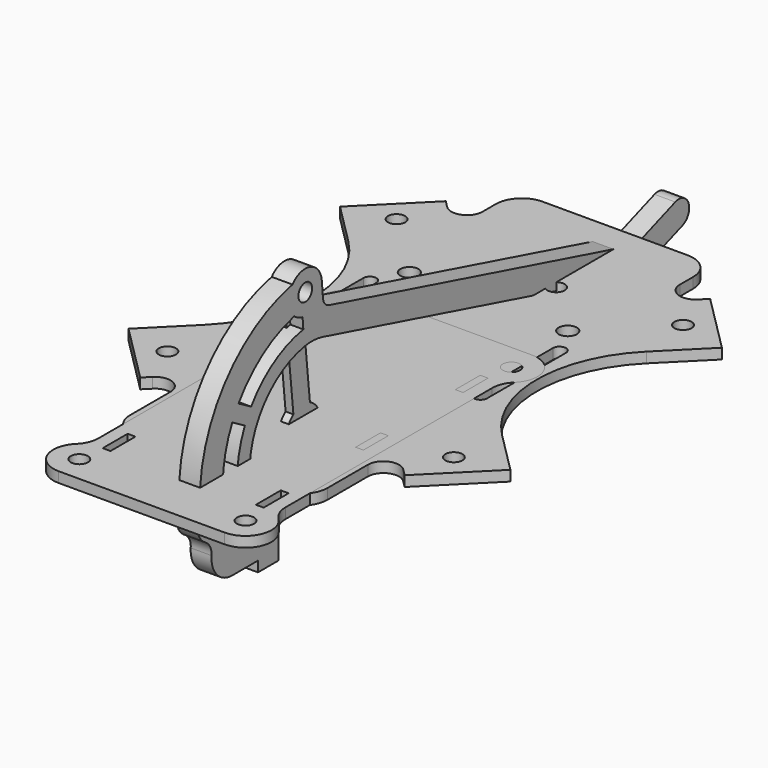
from build123d import *

# Parameters (mm, degrees)
F0_R      = 1.65
F1_DEPTH  = 4
F2_R      = 2
F3_R      = 1.65
F3_R_2    = 1.5
F4_DEPTH  = 1.5
F5_W      = 4
F5_H      = 5
F5_R      = 1.65
F5_R_2    = 1.75
F6_DEPTH  = 2
F7_R      = 1.5
F8_DEPTH  = 1.5
F9_R      = 1.65
F9_W      = 1.5
F9_H      = 6
F10_DEPTH = 2


with BuildPart() as f1:
    # F0 (on Right) → F1 (new body)
    with BuildSketch(Plane.YZ):
        with BuildLine():
            ThreePointArc((1.3715672107, 25.2116703552), (-1.4222724525, 28.6816418888), (-5.6933412888, 27.4150663864))
            ThreePointArc((-5.6933412888, 27.4150663864), (-22.1102697021, 17.1795219288), (-27.9717466489, -1.2575330657))
            ThreePointArc((-27.9717466489, -1.2575330657), (-28.0255548079, -1.9734585405), (-28.2479227846, -2.6560983329))
            ThreePointArc((-28.2479227846, -2.6560983329), (-28.4395274813, -5.5297709835), (-26.6511163601, -7.7872679434))
            ThreePointArc((-26.6511163601, -7.7872679434), (-25.5130767857, -8.9869520262), (-25.183571367, -10.607384731))
            ThreePointArc((-25.183571367, -10.607384731), (-23.8707312949, -14.3938859479), (-20.1990098767, -16))
            Line((-20.1990098767, -16), (-14, -16))
            Line((-14, -16), (-14, -18))
            Line((-14, -18), (-9, -18))
            Line((-9, -18), (-9, -16))
            Line((-9, -16), (-9, -13.7477270849))
            ThreePointArc((-9, -13.7477270849), (-9.1088672113, -13.2939844784), (-9.4117647059, -12.9390372563))
            ThreePointArc((-9.4117647059, -12.9390372563), (-11.0490391197, -11.5723262369), (-12.4899959968, -10))
            ThreePointArc((-12.4899959968, -10), (-14.9520494126, 5.6952803585), (-2.6721102867, 15.7752916491))
            ThreePointArc((-2.6721102867, 15.7752916491), (-0.5321831807, 15.9046899341), (1.5861490935, 15.5749926313))
            Line((1.5861490935, 15.5749926313), (77.2740661031, -4.7055236082))
            Line((77.2740661031, -4.7055236082), (88.1524135642, -0.7461289344))
            ThreePointArc((88.1524135642, -0.7461289344), (89.6465947578, 2.4581529759), (86.4423128475, 3.9523341695))
            Line((86.4423128475, 3.9523341695), (78.2305224207, 0.9634868841))
            ThreePointArc((78.2305224207, 0.9634868841), (77.0369193968, 0.726064481), (75.827165667, 0.8585540621))
            Line((75.827165667, 0.8585540621), (3.1187059905, 20.3407271153))
            ThreePointArc((3.1187059905, 20.3407271153), (2.1042551945, 20.9870035486), (1.6439546845, 22.0982672824))
            Line((1.6439546845, 22.0982672824), (1.3715672107, 25.2116703552))
        make_face()
        with Locations((-24.6201938253, -4.3412044417)):
            Circle(F0_R, mode=Mode.SUBTRACT)
        with BuildLine():
            Line((-16.1554944214, -10), (-20.1556443707, -10))
            ThreePointArc((-20.1556443707, -10), (-20.8662969598, -8.4171046796), (-21.4528611452, -6.7841542351))
            ThreePointArc((-21.4528611452, -6.7841542351), (-20.6244591351, -4.1565309852), (-21.6916970528, -1.6165197528))
            ThreePointArc((-21.6916970528, -1.6165197528), (-22.2990522616, -0.640297429), (-22.4946051617, 0.4926851121))
            ThreePointArc((-22.4946051617, 0.4926851121), (-21.8583588524, 5.3349928099), (-20.1922220952, 9.9259340546))
            Line((-20.1922220952, 9.9259340546), (-17.1531247023, 8.1713103568))
            ThreePointArc((-17.1531247023, 8.1713103568), (-18.97143002, -1.0415579663), (-16.1554944214, -10))
        make_face(mode=Mode.SUBTRACT)
        with BuildLine():
            ThreePointArc((-18.6922220952, 12.524010266), (-12.8614022088, 18.4616990882), (-5.2711524312, 21.8738417304))
            ThreePointArc((-5.2711524312, 21.8738417304), (-4.3390469936, 21.2545169172), (-3.2718535396, 20.9176461662))
            Line((-3.2718535396, 20.9176461662), (-3.0820652908, 18.7483565558))
            ThreePointArc((-3.0820652908, 18.7483565558), (-10.181739858, 16.0415764021), (-15.6531247023, 10.7693865681))
            Line((-15.6531247023, 10.7693865681), (-18.6922220952, 12.524010266))
        make_face(mode=Mode.SUBTRACT)
        with Locations((-2.6132115817, 24.8630473842)):
            Circle(F0_R, mode=Mode.SUBTRACT)
    extrude(amount=F1_DEPTH)

    # F2
    f2_edges = [f1.edges().sort_by_distance(p)[0] for p in [
        (2, -21.452861, -6.784154),
    ]]
    fillet(f2_edges, radius=F2_R)


with BuildPart() as f4:
    # F3 (on Right) → F4 (new body)
    with BuildSketch(Plane.YZ):
        with BuildLine():
            ThreePointArc((-5.4141735691, 26.9617641219), (-21.9624765263, 16.5499131367), (-27.4096595918, -2.2272317036))
            ThreePointArc((-27.4096595918, -2.2272317036), (-26.4229910161, -7.3411914898), (-21.444252554, -5.8120535302))
            Line((-21.444252554, -5.8120535302), (-3.0641777725, -2.5711504387))
            ThreePointArc((-3.0641777725, -2.5711504387), (3.1945420402, -2.4072600926), (1.6269465723, 3.6541818306))
            Line((1.6269465723, 3.6541818306), (-0.3239326382, 22.2155576451))
            ThreePointArc((-0.3239326382, 22.2155576451), (-0.2263571948, 27.4229157667), (-5.4141735691, 26.9617641219))
        make_face()
        with Locations((-24.6201938253, -4.3412044417)):
            Circle(F3_R, mode=Mode.SUBTRACT)
        Circle(F3_R_2, mode=Mode.SUBTRACT)
        with BuildLine():
            ThreePointArc((-22.9656262109, -1.2569855763), (-18.3686167311, 13.8417455325), (-5.1218923966, 22.4224489804))
            ThreePointArc((-5.1218923966, 22.4224489804), (-4.7350945422, 22.0795940072), (-4.3020202196, 21.797443792))
            Line((-4.3020202196, 21.797443792), (-2.3511410092, 3.2360679775))
            ThreePointArc((-2.3511410092, 3.2360679775), (-3.1945420402, 2.4072600926), (-3.7587704831, 1.3680805733))
            Line((-3.7587704831, 1.3680805733), (-22.1388452647, -1.8728225181))
            ThreePointArc((-22.1388452647, -1.8728225181), (-22.5294369202, -1.5342958996), (-22.9656262109, -1.2569855763))
        make_face(mode=Mode.SUBTRACT)
        with Locations((-2.6132115817, 24.8630473842)):
            Circle(F3_R, mode=Mode.SUBTRACT)
    extrude(amount=F4_DEPTH)


with BuildPart() as f6:
    # F5 (on Top) → F6 (new body)
    with BuildSketch(Plane.XY):
        with BuildLine():
            Line((14, 77), (-14, 77))
            ThreePointArc((-14, 77), (-17.5355339059, 75.5355339059), (-19, 72))
            Line((-19, 72), (-19, 68.8063491861))
            ThreePointArc((-19, 68.8063491861), (-20.8519497029, 66.0347105886), (-24.1213203436, 66.6850288425))
            Line((-24.1213203436, 66.6850288425), (-25.4558441227, 68.0195526217))
            Line((-25.4558441227, 68.0195526217), (-36.7695526217, 56.7058441227))
            Line((-36.7695526217, 56.7058441227), (-28.7027957955, 48.6390872965))
            ThreePointArc((-28.7027957955, 48.6390872965), (-21.5, 31.25), (-28.7027957955, 13.8609127035))
            Line((-28.7027957955, 13.8609127035), (-36.7695526217, 5.7941558773))
            Line((-36.7695526217, 5.7941558773), (-25.4558441227, -5.5195526217))
            Line((-25.4558441227, -5.5195526217), (-24.1213203436, -4.1850288425))
            ThreePointArc((-24.1213203436, -4.1850288425), (-20.8519497029, -3.5347105886), (-19, -6.3063491861))
            Line((-19, -6.3063491861), (-19, -16))
            ThreePointArc((-19, -16), (-17.5355339059, -19.5355339059), (-14, -21))
            Line((-14, -21), (-10, -21))
            ThreePointArc((-10, -21), (-9.1213203436, -18.8786796564), (-7, -18))
            Line((-7, -18), (7, -18))
            ThreePointArc((7, -18), (9.1213203436, -18.8786796564), (10, -21))
            Line((10, -21), (14, -21))
            ThreePointArc((14, -21), (17.5355339059, -19.5355339059), (19, -16))
            Line((19, -16), (19, -6.3063491861))
            ThreePointArc((19, -6.3063491861), (20.8519497029, -3.5347105886), (24.1213203436, -4.1850288425))
            Line((24.1213203436, -4.1850288425), (25.4558441227, -5.5195526217))
            Line((25.4558441227, -5.5195526217), (36.7695526217, 5.7941558773))
            Line((36.7695526217, 5.7941558773), (28.7027957955, 13.8609127035))
            ThreePointArc((28.7027957955, 13.8609127035), (21.5, 31.25), (28.7027957955, 48.6390872965))
            Line((28.7027957955, 48.6390872965), (36.7695526217, 56.7058441227))
            Line((36.7695526217, 56.7058441227), (25.4558441227, 68.0195526217))
            Line((25.4558441227, 68.0195526217), (24.1213203436, 66.6850288425))
            ThreePointArc((24.1213203436, 66.6850288425), (20.8519497029, 66.0347105886), (19, 68.8063491861))
            Line((19, 68.8063491861), (19, 72))
            ThreePointArc((19, 72), (17.5355339059, 75.5355339059), (14, 77))
        make_face()
        with Locations((-12, -11.5)):
            Rectangle(F5_W, F5_H, mode=Mode.SUBTRACT)
        with Locations((-6, -14)):
            Circle(F5_R, mode=Mode.SUBTRACT)
        with Locations((-27.5771644663, 3.6728355337)):
            Circle(F5_R, mode=Mode.SUBTRACT)
        with Locations((-5, 6)):
            Circle(F5_R, mode=Mode.SUBTRACT)
        with Locations((-15.25, 16)):
            Circle(F5_R_2, mode=Mode.SUBTRACT)
        with Locations((6, -14)):
            Circle(F5_R, mode=Mode.SUBTRACT)
        with Locations((12, -11.5)):
            Rectangle(F5_W, F5_H, mode=Mode.SUBTRACT)
        with Locations((5, 6)):
            Circle(F5_R, mode=Mode.SUBTRACT)
        with Locations((15.25, 16)):
            Circle(F5_R_2, mode=Mode.SUBTRACT)
        with Locations((27.5771644663, 3.6728355337)):
            Circle(F5_R, mode=Mode.SUBTRACT)
        with BuildLine():
            Line((-19.5, 21.75), (-19.5, 40.75))
            ThreePointArc((-19.5, 40.75), (-18.25, 42), (-17, 40.75))
            Line((-17, 40.75), (-17, 21.75))
            ThreePointArc((-17, 21.75), (-18.25, 20.5), (-19.5, 21.75))
        make_face(mode=Mode.SUBTRACT)
        with Locations((-15.25, 46.5)):
            Circle(F5_R_2, mode=Mode.SUBTRACT)
        with Locations((-27.5771644663, 58.8271644663)):
            Circle(F5_R, mode=Mode.SUBTRACT)
        with Locations((-5, 56.5)):
            Circle(F5_R, mode=Mode.SUBTRACT)
        with BuildLine():
            ThreePointArc((17, 40.75), (18.25, 42), (19.5, 40.75))
            Line((19.5, 40.75), (19.5, 21.75))
            ThreePointArc((19.5, 21.75), (18.25, 20.5), (17, 21.75))
            Line((17, 21.75), (17, 40.75))
        make_face(mode=Mode.SUBTRACT)
        with Locations((15.25, 46.5)):
            Circle(F5_R_2, mode=Mode.SUBTRACT)
        with Locations((5, 56.5)):
            Circle(F5_R, mode=Mode.SUBTRACT)
        with Locations((27.5771644663, 58.8271644663)):
            Circle(F5_R, mode=Mode.SUBTRACT)
    extrude(amount=F6_DEPTH)


with BuildPart() as f8:
    # F7 (on Top) → F8 (new body)
    with BuildSketch(Plane.XY):
        with BuildLine():
            Line((15.25, 18), (-15.25, 18))
            ThreePointArc((-15.25, 18), (-17.1945436483, 17.1945436483), (-18, 15.25))
            Line((-18, 15.25), (-18, -15.25))
            ThreePointArc((-18, -15.25), (-17.1945436483, -17.1945436483), (-15.25, -18))
            Line((-15.25, -18), (15.25, -18))
            ThreePointArc((15.25, -18), (17.1945436483, -17.1945436483), (18, -15.25))
            Line((18, -15.25), (18, 15.25))
            ThreePointArc((18, 15.25), (17.1945436483, 17.1945436483), (15.25, 18))
        make_face()
        with Locations((-15.25, -15.25)):
            Circle(F7_R, mode=Mode.SUBTRACT)
        with Locations((15.25, -15.25)):
            Circle(F7_R, mode=Mode.SUBTRACT)
        with Locations((-15.25, 15.25)):
            Circle(F7_R, mode=Mode.SUBTRACT)
        with Locations((15.25, 15.25)):
            Circle(F7_R, mode=Mode.SUBTRACT)
    extrude(amount=F8_DEPTH)


with BuildPart() as f10:
    # F9 (on Top) → F10 (new body)
    with BuildSketch(Plane.XY):
        with BuildLine():
            Line((16, 37), (-16, 37))
            ThreePointArc((-16, 37), (-20.6289075964, 33.8902948088), (-19.5, 28.4292857857))
            ThreePointArc((-19.5, 28.4292857857), (-18.3902277714, 26.7950632446), (-18, 24.8585715715))
            Line((-18, 24.8585715715), (-18, -24.8585715715))
            ThreePointArc((-18, -24.8585715715), (-18.3902277714, -26.7950632446), (-19.5, -28.4292857857))
            ThreePointArc((-19.5, -28.4292857857), (-20.6289075964, -33.8902948088), (-16, -37))
            Line((-16, -37), (16, -37))
            ThreePointArc((16, -37), (20.6289075964, -33.8902948088), (19.5, -28.4292857857))
            ThreePointArc((19.5, -28.4292857857), (18.3902277714, -26.7950632446), (18, -24.8585715715))
            Line((18, -24.8585715715), (18, 24.8585715715))
            ThreePointArc((18, 24.8585715715), (18.3902277714, 26.7950632446), (19.5, 28.4292857857))
            ThreePointArc((19.5, 28.4292857857), (20.6289075964, 33.8902948088), (16, 37))
        make_face()
        with Locations((-16, -32)):
            Circle(F9_R, mode=Mode.SUBTRACT)
        with Locations((-14.75, -24)):
            Rectangle(F9_W, F9_H, mode=Mode.SUBTRACT)
        with Locations((16, -32)):
            Circle(F9_R, mode=Mode.SUBTRACT)
        with Locations((14.75, -24)):
            Rectangle(F9_W, F9_H, mode=Mode.SUBTRACT)
        with Locations((-14.75, 0)):
            Rectangle(F9_W, F9_H, mode=Mode.SUBTRACT)
        with Locations((-14.75, 24)):
            Rectangle(F9_W, F9_H, mode=Mode.SUBTRACT)
        with Locations((-16, 32)):
            Circle(F9_R, mode=Mode.SUBTRACT)
        with Locations((14.75, 0)):
            Rectangle(F9_W, F9_H, mode=Mode.SUBTRACT)
        with Locations((14.75, 24)):
            Rectangle(F9_W, F9_H, mode=Mode.SUBTRACT)
        with Locations((16, 32)):
            Circle(F9_R, mode=Mode.SUBTRACT)
    extrude(amount=F10_DEPTH)


solid = Compound([f1.part, f4.part, f6.part, f8.part, f10.part])
